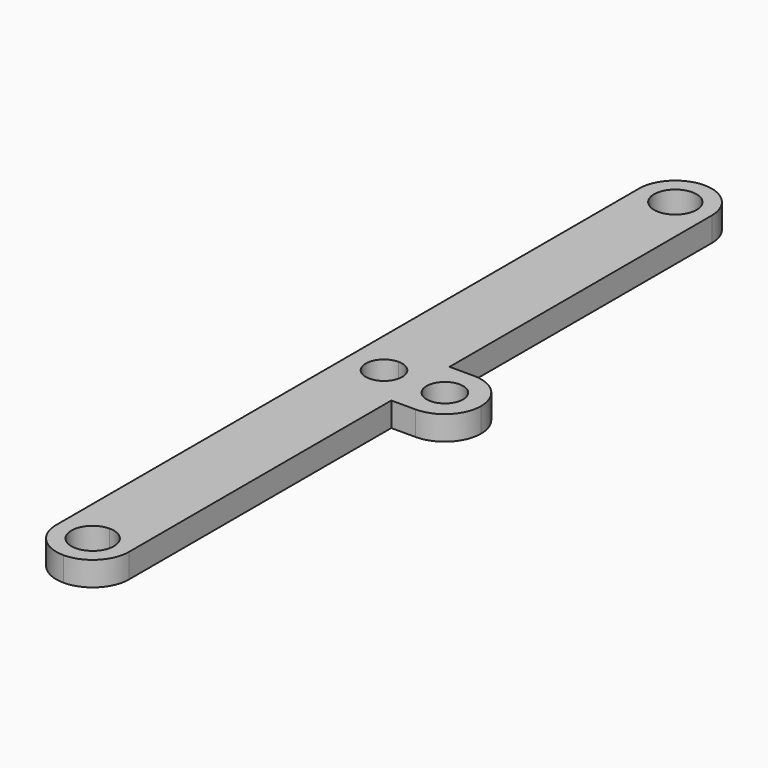
from build123d import *

# Parameters (mm, degrees)
F0_W     = 6
F0_H     = 66
F1_DEPTH = 2
F3_DEPTH = 2
F5_DEPTH = 5
F6_R     = 1.5
F7_DEPTH = 2
F8_R     = 2.99999


# Not quite as in the source:
# - a fillet or chamfer is up to 0.001 mm smaller than in the source, because OpenCascade refuses the exact size


with BuildPart() as f1:
    # F0 (on Top) → F1 (new body)
    with BuildSketch(Plane.XY):
        Rectangle(F0_W, F0_H)
    extrude(amount=F1_DEPTH)

    # F2 (on face) → F3 (cut, through all)
    with BuildSketch(Plane.XY.offset(2)):
        with BuildLine():
            ThreePointArc((0, -1.5), (1.0606601718, -1.0606601718), (1.5, 0))
            ThreePointArc((1.5, 0), (1.0606601718, 1.0606601718), (0, 1.5))
            Line((0, 1.5), (0, 0))
            Line((0, 0), (0, -1.5))
        make_face()
        with BuildLine():
            ThreePointArc((1.75, -30), (1.2374368671, -28.7625631329), (0, -28.25))
            ThreePointArc((0, -28.25), (-1.2374368671, -31.2374368671), (1.75, -30))
        make_face()
        with BuildLine():
            ThreePointArc((1.75, 30), (-1.2374368671, 31.2374368671), (0, 28.25))
            ThreePointArc((0, 28.25), (1.2374368671, 28.7625631329), (1.75, 30))
        make_face()
        with BuildLine():
            Line((0, 0), (0, 1.5))
            ThreePointArc((0, 1.5), (-1.5, 0), (0, -1.5))
            Line((0, -1.5), (0, 0))
        make_face()
    extrude(amount=-F3_DEPTH, mode=Mode.SUBTRACT)

    # F4 (on face) → F5 (join)
    with BuildSketch(Plane.YZ.offset(3)):
        Polygon((3, 2), (0, 2), (-3, 2), (-3, 0), (0, 0), (3, 0), align=None)
    extrude(amount=F5_DEPTH)

    # F6 (on face) → F7 (cut, through all)
    with BuildSketch(Plane.XY.offset(2)):
        with Locations((5.0139404441, 0)):
            Circle(F6_R)
    extrude(amount=-F7_DEPTH, mode=Mode.SUBTRACT)

    # F8 (radius 3 in the source; OpenCascade refuses exactly that, so slightly less here)
    f8_edges = [f1.edges().sort_by_distance(p)[0] for p in [
        (-3, -33, 1),
        (3, -33, 1),
        (3, 33, 1),
        (-3, 33, 1),
        (8, -3, 1),
        (8, 3, 1),
    ]]
    fillet(f8_edges, radius=F8_R)


solid = f1.part
